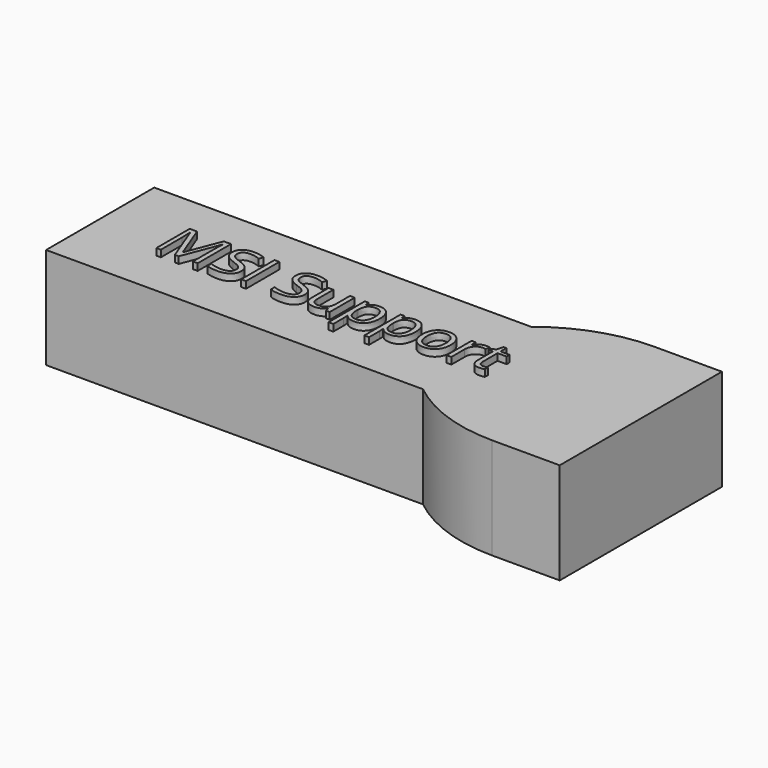
from build123d import *

# Parameters (mm, degrees)
F1_DEPTH     = 15
F2_TEXT_SIZE = 8.6388423951
F3_DEPTH     = 16


# Not quite as in the source:
# - Text() gives the source's letters only with a copy of the font that has no kerning and outlines rounded to 1/6400 em; it was checked with that copy


with BuildPart() as f1:
    # F0 (on Top) → F1 (new body)
    with BuildSketch(Plane.XY):
        Polygon((20.7662303001, 10), (-35, 10), (-35, -10), (20.7662303001, -10), (35, -10), (35, 10), align=None)
        with BuildLine():
            ThreePointArc((35, 15), (27.4567878216, 13.7136490018), (20.7662303001, 10))
            Line((20.7662303001, 10), (35, 10))
            Line((35, 10), (35, 15))
        make_face()
        Polygon((35, 15), (35, 10), (35, -10), (35, -15), (45, -15), (45, 15), align=None)
        with BuildLine():
            Line((35, -10), (20.7662303001, -10))
            ThreePointArc((20.7662303001, -10), (27.4567878216, -13.7136490018), (35, -15))
            Line((35, -15), (35, -10))
        make_face()
    extrude(amount=F1_DEPTH)

    # F2 (on Top) → F3 (join)
    with BuildSketch(Plane.XY):
        with Locations((-25, -3.1573261622)):
            Text('MSI Support', F2_TEXT_SIZE, font='Open Sans', text_align=(TextAlign.LEFT, TextAlign.BOTTOM))
    extrude(amount=F3_DEPTH)


solid = f1.part
